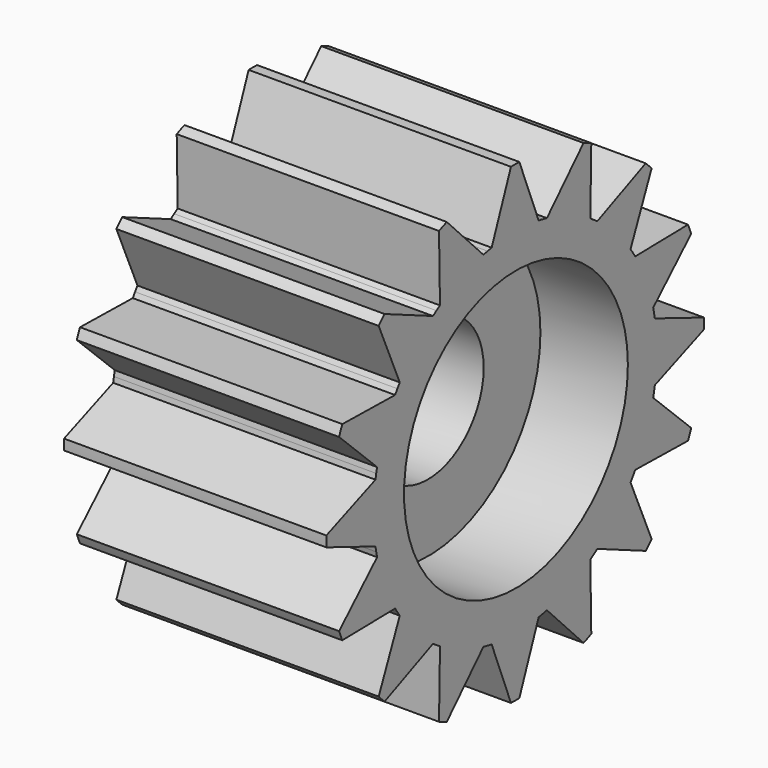
from build123d import *

# Parameters (mm, degrees)
F0_R            = 13.5
F1_DEPTH        = 15
F2_R            = 7
F3_DEPTH        = 5
F5_DEPTH        = 15.001
F5_COPIES_COUNT = 16
F6_R            = 8
F7_DEPTH        = 5
F8_R            = 4
F9_DEPTH        = 10.001


# Not quite as in the source:
# - a pattern or mirror of a feature is missing from the dataset's text; its kind, count and spacing are read off the source's solid


with BuildPart() as f1:
    # F0 (on Right) → F1 (new body)
    with BuildSketch(Plane.YZ):
        Circle(F0_R)
    extrude(amount=-F1_DEPTH)

    # F2 (on face) → F3 (cut)
    with BuildSketch(Plane(origin=(-15, 0, 0), x_dir=(0, -1, 0), z_dir=(-1, 0, 0))):
        Circle(F2_R)
    extrude(amount=-F3_DEPTH, mode=Mode.SUBTRACT)

    # F4 (on face) → F5 (cut, through all)
    with BuildSketch(Plane(origin=(-15, 0, 0), x_dir=(0, -1, 0), z_dir=(-1, 0, 0))):
        with BuildLine():
            Line((2.2686257354, 9.8675712449), (4.8878039751, 12.5840920332))
            ThreePointArc((4.8878039751, 12.5840920332), (2.6337193472, 13.2406012854), (0.2999814809, 13.4966666667))
            Line((0.2999814809, 13.4966666667), (1.6802191492, 9.9846125919))
            Line((1.6802191492, 9.9846125919), (1.9752895104, 9.9304509641))
            Line((1.9752895104, 9.9304509641), (2.2686257354, 9.8675712449))
        make_face()
    f5 = extrude(amount=-F5_DEPTH, mode=Mode.SUBTRACT)

    # F5_copies: F5 ×16 about axis
    f5_copies_axis = Axis((0, 0, 0), (1, 0, 0))
    for i in range(1, F5_COPIES_COUNT):
        add(f5.rotate(f5_copies_axis, i * 360 / F5_COPIES_COUNT), mode=Mode.SUBTRACT)

    # F6 (on face) → F7 (cut)
    with BuildSketch(Plane.YZ):
        with Locations((0.0570340926, 0.13036374)):
            Circle(F6_R)
    extrude(amount=-F7_DEPTH, mode=Mode.SUBTRACT)

    # F8 (on face) → F9 (cut, through all)
    with BuildSketch(Plane.YZ.offset(-5)):
        Circle(F8_R)
    extrude(amount=-F9_DEPTH, mode=Mode.SUBTRACT)


solid = f1.part
